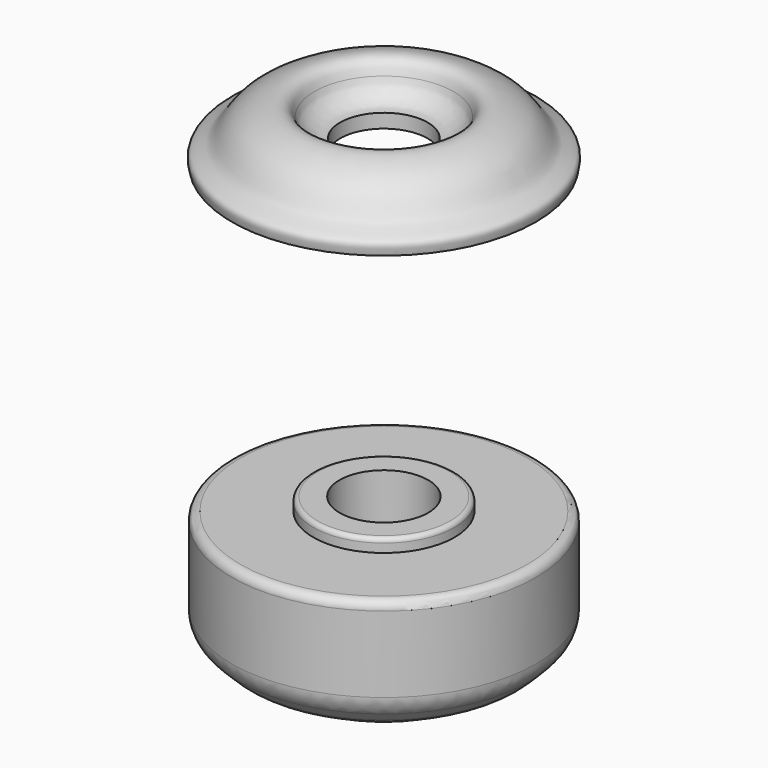
from build123d import *

# Parameters (mm, degrees)
F0_R      = 17.5438891732
F1_DEPTH  = 14
F2_R      = 12.0120819091
F3_DEPTH  = 1.5
F4_R      = 8.1414232705
F5_DEPTH  = 1.5
F6_R      = 5.1023864689
F7_DEPTH  = 25
F8_SIZE   = 3
F9_R      = 3
F10_R     = 1
F11_R     = 0.5
F14_R     = 3
F16_R     = 5.0286050309
F17_DEPTH = 20


# Not quite as in the source:
# - a fillet or chamfer that OpenCascade refuses, or shapes differently, is made with other operations: its cross-section is extruded or revolved along the edge and cut away or added


with BuildPart() as f1:
    # F0 (on Top) → F1 (new body)
    with BuildSketch(Plane.XY):
        Circle(F0_R)
    extrude(amount=F1_DEPTH)

    # F2 (on face) → F3 (join)
    with BuildSketch(Plane(origin=(0, 0, 0), x_dir=(1, 0, 0), z_dir=(0, 0, -1))):
        Circle(F2_R)
    extrude(amount=F3_DEPTH)

    # F4 (on face) → F5 (join)
    with BuildSketch(Plane.XY.offset(14)):
        Circle(F4_R)
    extrude(amount=F5_DEPTH)

    # F6 (on face) → F7 (cut)
    with BuildSketch(Plane.XY.offset(15.5)):
        Circle(F6_R)
    extrude(amount=-F7_DEPTH, mode=Mode.SUBTRACT)

    # F8
    f8_edges = [f1.edges().sort_by_distance(p)[0] for p in [
        (-17.543889, 0, 0),
    ]]
    chamfer(f8_edges, length=F8_SIZE)

    # F9
    f9_edges = [f1.edges().sort_by_distance(p)[0] for p in [
        (16.043889, 0, 1.5),
        (-17.543889, 0, 3),
        (-14.543889, 0, 0),
    ]]
    fillet(f9_edges, radius=F9_R)

    # F10
    f10_edges = [f1.edges().sort_by_distance(p)[0] for p in [
        (-17.543889, 0, 14),
        (-12.012082, 0, -1.5),
    ]]
    fillet(f10_edges, radius=F10_R)

    # F11
    f11_edges = [f1.edges().sort_by_distance(p)[0] for p in [
        (-8.141423, 0, 15.5),
    ]]
    fillet(f11_edges, radius=F11_R)


with BuildPart() as f13:
    # F12 (on Front) → F13 (revolve)
    with BuildSketch(Plane.XZ):
        with BuildLine():
            Line((7.655496709, 51.7671853304), (0, 51.7671853304))
            Line((0, 51.7671853304), (0, 50.1541830599))
            Line((0, 50.1541830599), (8.6348215118, 50.1541830599))
            Line((8.6348215118, 50.1541830599), (9.0956799686, 51.9400089979))
            Line((9.0956799686, 51.9400089979), (11.1695425585, 53.2649755478))
            Line((11.1695425585, 53.2649755478), (13.2434051484, 51.536757499))
            Line((13.2434051484, 51.536757499), (15.4900895432, 49.5781078935))
            Line((15.4900895432, 49.5781078935), (17.5, 49.0020364523))
            add(Edge.make_bspline(
                [(7.655496709, 51.7671853304), (7.8052236894, 53.3355937889), (8.1289722473, 56.7268995876), (14.497666046, 54.0315890321), (15.2829429137, 51.0603268241), (17.9005469417, 50.6214675024), (17.6245672577, 49.5056680221), (17.5, 49.0020364523)],
                knots=[0, 0, 0, 0, 0.229104146, 0.4953825737, 0.6995885707, 0.8644051351, 1, 1, 1, 1], degree=3))
        make_face()
    revolve(axis=Axis((0, 0, 53.6106191576), (0, 0, -1)))

    # F14
    f14_edges = [f13.edges().sort_by_distance(p)[0] for p in [
        (-7.655497, 0, 51.767185),
    ]]
    fillet(f14_edges, radius=F14_R)

    # F15: fillet of radius 5 on 1 edges, made by hand

    # F15_s1 → F15_t2 (revolve, cut)
    with BuildSketch(Plane.XZ):
        with BuildLine():
            ThreePointArc((9.0956799686, 51.9400089979), (7.3786074945, 50.6225790222), (5.2656558043, 50.1541830599))
            Line((5.2656558043, 50.1541830599), (5.2656558043, 50.0541830599))
            Line((5.2656558043, 50.0541830599), (8.6348215118, 50.0541830599))
            Line((8.6348215118, 50.0541830599), (8.7316492422, 50.1291952504))
            ThreePointArc((8.7316492422, 50.1291952504), (8.9620784706, 51.0221082194), (9.1722804519, 51.8757255167))
            Line((9.1722804519, 51.8757255167), (9.0956799686, 51.9400089979))
        make_face()
    revolve(axis=Axis((0, 0, 50.1541830599), (0, 0, -1)), mode=Mode.SUBTRACT)

    # F16 (on face) → F17 (cut)
    with BuildSketch(Plane.XY.offset(51.7671853304)):
        Circle(F16_R)
    extrude(amount=-F17_DEPTH, mode=Mode.SUBTRACT)


solid = Compound([f1.part, f13.part])
